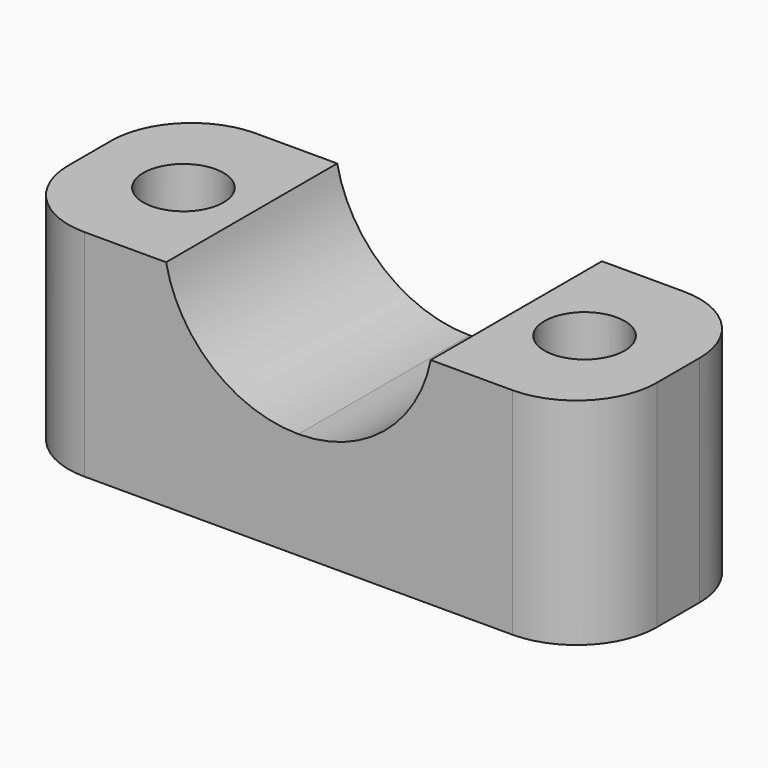
from build123d import *

# Parameters (mm, degrees)
F1_DEPTH = 8
F2_R     = 1.5
F3_DEPTH = 25
F4_R     = 3


# Not quite as in the source:
# - a pattern or mirror of a feature is missing from the dataset's text; its kind, count and spacing are read off the source's solid


with BuildPart() as f1:
    # F0 (on Front) → F1 (new body)
    with BuildSketch(Plane.XZ):
        with BuildLine():
            Line((11, 0), (11, 8.05))
            Line((11, 8.05), (4.95, 8.05))
            ThreePointArc((4.95, 8.05), (3.1978508408, 5.141515639), (0, 4))
            Line((0, 4), (0, 0))
            Line((0, 0), (11, 0))
        make_face()
    extrude(amount=F1_DEPTH)

    # F1_copies: F1 across plane


with BuildPart() as f1_1:
    add(f1.part)
    add(f1.part.mirror(Plane(origin=(0, 0, 0), x_dir=(0, 0, -1), z_dir=(-1, 0, 0))))

    # F2 (on face) → F3 (cut)
    with BuildSketch(Plane.XY.offset(8.05)):
        with Locations((7.5, -4)):
            Circle(F2_R)
    f3 = extrude(amount=-F3_DEPTH, mode=Mode.SUBTRACT)

    # F3_copies: F3 across plane
    add(f3.mirror(Plane(origin=(0, 0, 0), x_dir=(0, 0, -1), z_dir=(-1, 0, 0))), mode=Mode.SUBTRACT)

    # F4
    f4_edges = [f1_1.edges().sort_by_distance(p)[0] for p in [
        (11, 0, 4.025),
        (11, -8, 4.025),
        (-11, 0, 4.025),
        (-11, -8, 4.025),
    ]]
    fillet(f4_edges, radius=F4_R)


solid = f1_1.part
